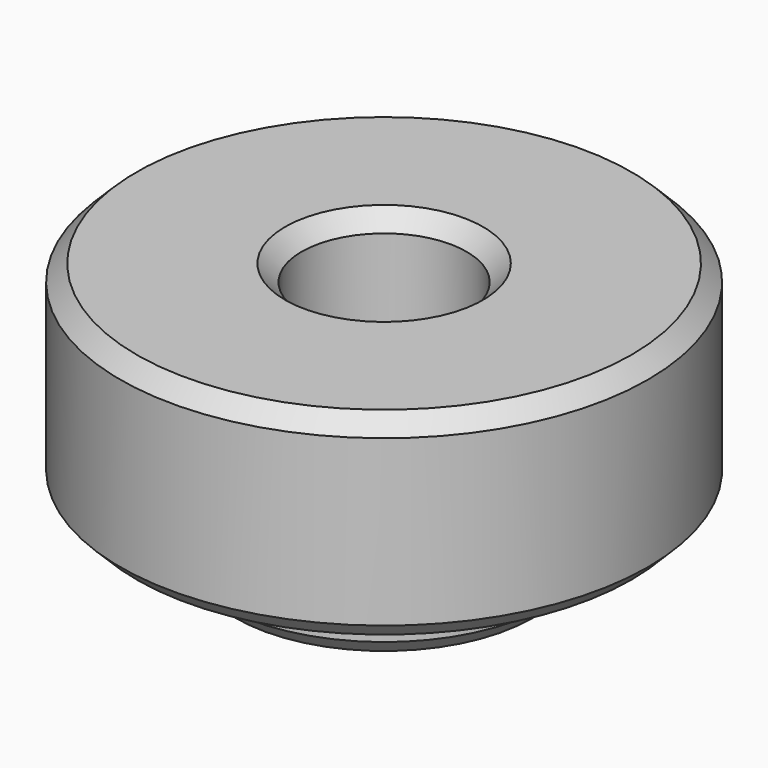
from build123d import *

# Parameters (mm, degrees)
F0_R     = 4
F1_DEPTH = 3
F2_R     = 2.5
F3_DEPTH = 1
F5_D     = 2.5
F6_SIZE  = 0.25


with BuildPart() as f1:
    # F0 (on Top) → F1 (new body)
    with BuildSketch(Plane.XY):
        Circle(F0_R)
    extrude(amount=-F1_DEPTH)

    # F2 (on face) → F3 (join)
    with BuildSketch(Plane(origin=(0, 0, -3), x_dir=(1, 0, 0), z_dir=(0, 0, -1))):
        Circle(F2_R)
    extrude(amount=F3_DEPTH)

    # F5 (through all)
    with Locations(Plane.XY):
        with Locations((0, 0)):
            Hole(F5_D / 2)

    # F6
    f6_edges = [f1.edges().sort_by_distance(p)[0] for p in [
        (-4, 0, 0),
        (-4, 0, -3),
        (-2.5, 0, -4),
        (-1.25, 0, 0),
    ]]
    chamfer(f6_edges, length=F6_SIZE)


solid = f1.part
